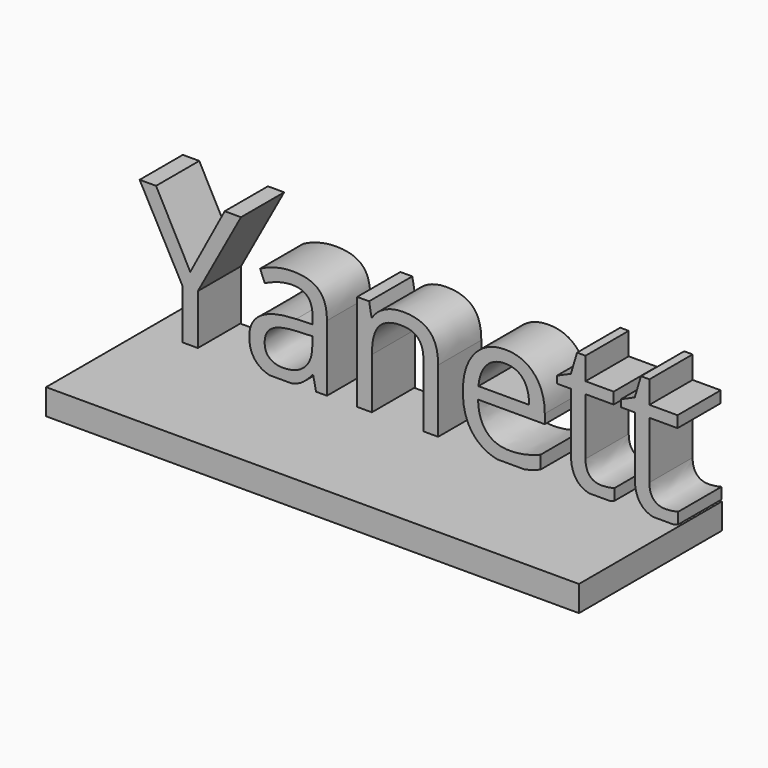
from build123d import *

# Parameters (mm, degrees)
F0_TEXT_SIZE = 85.1425368132
F1_DEPTH     = 25.4
F2_W         = 250.6788149476
F2_H         = 12.0878387243
F3_DEPTH     = 84.074


# Not quite as in the source:
# - Text() gives the source's letters only with a copy of the font that has no kerning and outlines rounded to 1/6400 em; it was checked with that copy


with BuildPart() as f1:
    # F0 (on Front) → F1 (new body)
    with BuildSketch(Plane.XZ):
        with Locations((-123.3345968649, -23.6000735313)):
            Text('Yanett', F0_TEXT_SIZE, font='Open Sans', text_align=(TextAlign.LEFT, TextAlign.BOTTOM))
    extrude(amount=F1_DEPTH)


with BuildPart() as f3:
    # F2 (on Front) → F3 (new body)
    with BuildSketch(Plane.XZ):
        with Locations((4.9377642572, -29.931797646)):
            Rectangle(F2_W, F2_H)
    extrude(amount=F3_DEPTH)


solid = Compound([f1.part, f3.part])
